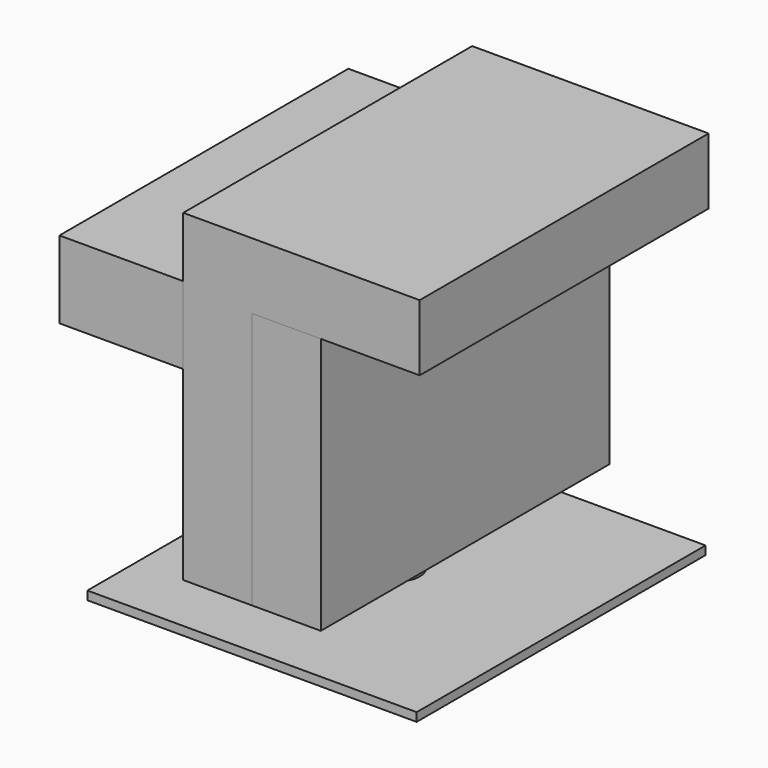
from build123d import *

# Parameters (mm, degrees)
F2_DEPTH      = 210
F2_DEPTH_BACK = 210
F1_W          = 80
F1_H          = 299
F3_DEPTH      = 210
F3_DEPTH_BACK = 210
F1_W_2        = 144
F1_H_2        = 90
F4_W          = 27
F4_H          = 47
F5_W          = 383
F5_H          = 10
F7_DEPTH      = 210
F7_DEPTH_BACK = 210


with BuildPart() as f2:
    # F0 (on Front) → F2 (new body, two sides)
    with BuildSketch(Plane.XZ) as f2_sk:
        Polygon((195, 188), (-80, 188), (-80, -188), (0, -188), (0, 111), (195, 111), align=None)
    extrude(amount=F2_DEPTH)
    extrude(f2_sk.sketch, amount=-F2_DEPTH_BACK)


with BuildPart() as f3:
    # F1 (on Front) → F3 (new body, two sides)
    with BuildSketch(Plane.XZ) as f3_sk:
        with Locations((40, -38.5)):
            Rectangle(F1_W, F1_H)
    extrude(amount=F3_DEPTH)
    extrude(f3_sk.sketch, amount=-F3_DEPTH_BACK)


with BuildPart() as f3b:
    # F1 (on Front) → F3, piece 2 (new body, two sides)
    with BuildSketch(Plane.XZ) as f3_2_sk:
        with Locations((-152, 73)):
            Rectangle(F1_W_2, F1_H_2)
    extrude(amount=F3_DEPTH)
    extrude(f3_2_sk.sketch, amount=-F3_DEPTH_BACK)


with BuildPart() as f6:
    # F4 (on Front) → F6 (revolve)
    with BuildSketch(Plane.XZ):
        with Locations((-13.5, -211.5)):
            Rectangle(F4_W, F4_H)
    revolve(axis=Axis((0, 0, -211.5), (0, 0, 1)))


with BuildPart() as f7:
    # F5 (on Front) → F7 (new body, two sides)
    with BuildSketch(Plane.XZ) as f7_sk:
        with Locations((0, -240)):
            Rectangle(F5_W, F5_H)
    extrude(amount=F7_DEPTH)
    extrude(f7_sk.sketch, amount=-F7_DEPTH_BACK)


solid = Compound([f2.part, f3.part, f3b.part, f6.part, f7.part])
